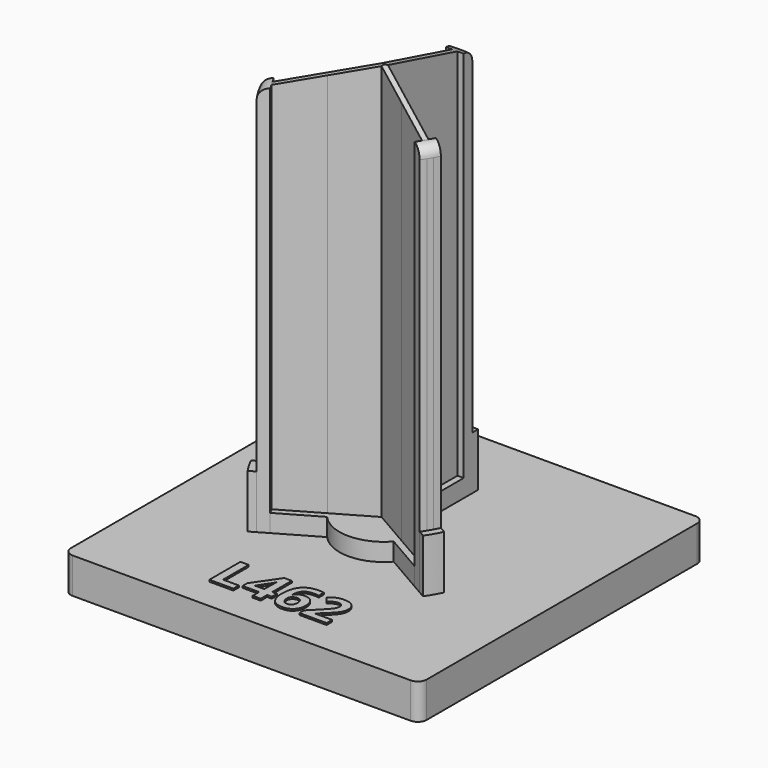
from build123d import *

# Parameters (mm, degrees)
F0_R         = 3.5
F0_R_2       = 1.75
F1_DEPTH     = 10
F2_DEPTH     = 220
F3_DEPTH     = 235
F4_T4_DEPTH  = 293.7329049929
F4_T9_DEPTH  = 293.7329049929
F4_T14_DEPTH = 293.7329049929
F5_T2_ANGLE  = 40.9393595263
F5_T4_ANGLE  = 40.9393595263
F5_T6_ANGLE  = 40.9393595263
F6_DEPTH     = 3
F7_DEPTH     = 30
F8_W         = 200
F8_H         = 200
F9_DEPTH     = 20
F10_R        = 5
F0_TEXT_SIZE = 30.5555555556
F11_DEPTH    = 1


# Not quite as in the source:
# - a fillet or chamfer that OpenCascade refuses, or shapes differently, is made with other operations: its cross-section is extruded or revolved along the edge and cut away or added
# - a feature names something its author has since deleted; it is built from what else it names
# - Text() gives the source's letters only with a copy of the font that has no kerning and outlines rounded to 1/6400 em; it was checked with that copy


with BuildPart() as f1:
    # F0 (on Top) → F1 (new body)
    with BuildSketch(Plane.XY):
        with BuildLine():
            ThreePointArc((25, 0), (19.364916731, 15.8113883008), (5, 24.4948974278))
            ThreePointArc((5, 24.4948974278), (3.2581304855, 24.7867824806), (1.5, 24.9549594269))
            Line((1.5, 24.9549594269), (1.5, 0.8660254038))
            Line((1.5, 0.8660254038), (22.3616288141, -11.1784416078))
            ThreePointArc((22.3616288141, -11.1784416078), (23.095048549, -9.571767471), (23.7132034356, -7.917321695))
            ThreePointArc((23.7132034356, -7.917321695), (24.6762039817, -4.0106055721), (25, 0))
        make_face()
        with Locations((11.9308144071, 6.8882589096)):
            Circle(F0_R, mode=Mode.SUBTRACT)
        with BuildLine():
            Line((5, 24.4948974278), (5, 49.7493718553))
            Line((5, 49.7493718553), (1.5, 49.7493718553))
            Line((1.5, 49.7493718553), (1.5, 24.9549594269))
            ThreePointArc((1.5, 24.9549594269), (3.2581304855, 24.7867824806), (5, 24.4948974278))
        make_face()
        with BuildLine():
            Line((43.834219849, -23.575647822), (45.584219849, -20.5445589087))
            Line((45.584219849, -20.5445589087), (23.7132034356, -7.917321695))
            ThreePointArc((23.7132034356, -7.917321695), (23.095048549, -9.571767471), (22.3616288141, -11.1784416078))
            Line((22.3616288141, -11.1784416078), (43.834219849, -23.575647822))
        make_face()
        with Locations((11.9308144071, 6.8882589096)):
            Circle(F0_R)
        with Locations((11.9308144071, 6.8882589096)):
            Circle(F0_R_2, mode=Mode.SUBTRACT)
        with Locations((11.9308144071, 6.8882589096)):
            Circle(F0_R_2)
    extrude(amount=F1_DEPTH)



with BuildPart() as f1b:
    # F0 (on Top) → F1, piece 2 (new body)
    with BuildSketch(Plane.XY):
        with BuildLine():
            Line((-1.5, 49.7493718553), (-5, 49.7493718553))
            Line((-5, 49.7493718553), (-5, 24.4948974278))
            ThreePointArc((-5, 24.4948974278), (-3.2581304855, 24.7867824806), (-1.5, 24.9549594269))
            Line((-1.5, 24.9549594269), (-1.5, 49.7493718553))
        make_face()
        with BuildLine():
            Line((-23.7132034356, -7.917321695), (-45.584219849, -20.5445589087))
            Line((-45.584219849, -20.5445589087), (-43.834219849, -23.575647822))
            Line((-43.834219849, -23.575647822), (-22.3616288141, -11.1784416078))
            ThreePointArc((-22.3616288141, -11.1784416078), (-23.095048549, -9.571767471), (-23.7132034356, -7.917321695))
        make_face()
        with BuildLine():
            ThreePointArc((-1.5, 24.9549594269), (-3.2581304855, 24.7867824806), (-5, 24.4948974278))
            ThreePointArc((-5, 24.4948974278), (-21.6506350946, 12.5), (-23.7132034356, -7.917321695))
            ThreePointArc((-23.7132034356, -7.917321695), (-23.095048549, -9.571767471), (-22.3616288141, -11.1784416078))
            Line((-22.3616288141, -11.1784416078), (-1.5, 0.8660254038))
            Line((-1.5, 0.8660254038), (-1.5, 24.9549594269))
        make_face()
        with Locations((-11.9308144071, 6.8882589096)):
            Circle(F0_R, mode=Mode.SUBTRACT)
        with Locations((-11.9308144071, 6.8882589096)):
            Circle(F0_R)
        with Locations((-11.9308144071, 6.8882589096)):
            Circle(F0_R_2, mode=Mode.SUBTRACT)
        with Locations((-11.9308144071, 6.8882589096)):
            Circle(F0_R_2)
    extrude(amount=F1_DEPTH)


with BuildPart() as f1c:
    # F0 (on Top) → F1, piece 3 (new body)
    with BuildSketch(Plane.XY):
        with BuildLine():
            ThreePointArc((-18.7132034356, -16.5775757328), (0, -25), (18.7132034356, -16.5775757328))
            ThreePointArc((18.7132034356, -16.5775757328), (19.8369180635, -15.2150150096), (20.8616288141, -13.7765178191))
            Line((20.8616288141, -13.7765178191), (0, -1.7320508076))
            Line((0, -1.7320508076), (-20.8616288141, -13.7765178191))
            ThreePointArc((-20.8616288141, -13.7765178191), (-19.8369180635, -15.2150150096), (-18.7132034356, -16.5775757328))
        make_face()
        with Locations((0, -13.7765178191)):
            Circle(F0_R, mode=Mode.SUBTRACT)
        with BuildLine():
            Line((18.7132034356, -16.5775757328), (40.584219849, -29.2048129466))
            Line((40.584219849, -29.2048129466), (42.334219849, -26.1737240333))
            Line((42.334219849, -26.1737240333), (20.8616288141, -13.7765178191))
            ThreePointArc((20.8616288141, -13.7765178191), (19.8369180635, -15.2150150096), (18.7132034356, -16.5775757328))
        make_face()
        with BuildLine():
            Line((-42.334219849, -26.1737240333), (-40.584219849, -29.2048129466))
            Line((-40.584219849, -29.2048129466), (-18.7132034356, -16.5775757328))
            ThreePointArc((-18.7132034356, -16.5775757328), (-19.8369180635, -15.2150150096), (-20.8616288141, -13.7765178191))
            Line((-20.8616288141, -13.7765178191), (-42.334219849, -26.1737240333))
        make_face()
        with Locations((0, -13.7765178191)):
            Circle(F0_R)
        with Locations((0, -13.7765178191)):
            Circle(F0_R_2, mode=Mode.SUBTRACT)
        with Locations((0, -13.7765178191)):
            Circle(F0_R_2)
    extrude(amount=F1_DEPTH)


with BuildPart() as f1_1:
    add(f1.part)

    add(f1b.part)  # F2 merges F1b

    add(f1c.part)  # F2 merges F1c
    # F0 (on Top) → F2 (join)
    with BuildSketch(Plane.XY):
        with BuildLine():
            Line((5, 49.7493718553), (5, 55.7763390695))
            ThreePointArc((5, 55.7763390695), (3.2515934535, 55.9055197634), (1.5, 55.9799071096))
            Line((1.5, 55.9799071096), (1.5, 49.7493718553))
            Line((1.5, 49.7493718553), (5, 49.7493718553))
        make_face()
        with BuildLine():
            ThreePointArc((-1.5, 55.9799071096), (-3.2515934535, 55.9055197634), (-5, 55.7763390695))
            Line((-5, 55.7763390695), (-5, 49.7493718553))
            Line((-5, 49.7493718553), (-1.5, 49.7493718553))
            Line((-1.5, 49.7493718553), (-1.5, 55.9799071096))
        make_face()
        with BuildLine():
            ThreePointArc((-47.7300216584, -29.2889916605), (-46.7898036001, -30.7687224152), (-45.8037265643, -32.2182965537))
            Line((-45.8037265643, -32.2182965537), (-40.584219849, -29.2048129466))
            Line((-40.584219849, -29.2048129466), (-42.334219849, -26.1737240333))
            Line((-42.334219849, -26.1737240333), (-47.7300216584, -29.2889916605))
        make_face()
        with BuildLine():
            Line((-45.584219849, -20.5445589087), (-50.8037265643, -23.5580425158))
            ThreePointArc((-50.8037265643, -23.5580425158), (-50.0413970536, -25.1367973482), (-49.2300216584, -26.6909154491))
            Line((-49.2300216584, -26.6909154491), (-43.834219849, -23.575647822))
            Line((-43.834219849, -23.575647822), (-45.584219849, -20.5445589087))
        make_face()
        with BuildLine():
            Line((40.584219849, -29.2048129466), (45.8037265643, -32.2182965537))
            ThreePointArc((45.8037265643, -32.2182965537), (46.7898036001, -30.7687224152), (47.7300216584, -29.2889916605))
            Line((47.7300216584, -29.2889916605), (42.334219849, -26.1737240333))
            Line((42.334219849, -26.1737240333), (40.584219849, -29.2048129466))
        make_face()
        with BuildLine():
            ThreePointArc((49.2300216584, -26.6909154491), (50.0413970536, -25.1367973482), (50.8037265643, -23.5580425158))
            Line((50.8037265643, -23.5580425158), (45.584219849, -20.5445589087))
            Line((45.584219849, -20.5445589087), (43.834219849, -23.575647822))
            Line((43.834219849, -23.575647822), (49.2300216584, -26.6909154491))
        make_face()
        with BuildLine():
            Line((-43.834219849, -23.575647822), (-49.2300216584, -26.6909154491))
            ThreePointArc((-49.2300216584, -26.6909154491), (-48.4974226119, -28), (-47.7300216584, -29.2889916605))
            Line((-47.7300216584, -29.2889916605), (-42.334219849, -26.1737240333))
            Line((-42.334219849, -26.1737240333), (-43.834219849, -23.575647822))
        make_face()
        with BuildLine():
            ThreePointArc((47.7300216584, -29.2889916605), (48.4974226119, -28), (49.2300216584, -26.6909154491))
            Line((49.2300216584, -26.6909154491), (43.834219849, -23.575647822))
            Line((43.834219849, -23.575647822), (42.334219849, -26.1737240333))
            Line((42.334219849, -26.1737240333), (47.7300216584, -29.2889916605))
        make_face()
        with BuildLine():
            Line((1.5, 49.7493718553), (1.5, 55.9799071096))
            ThreePointArc((1.5, 55.9799071096), (0, 56), (-1.5, 55.9799071096))
            Line((-1.5, 55.9799071096), (-1.5, 49.7493718553))
            Line((-1.5, 49.7493718553), (1.5, 49.7493718553))
        make_face()
    extrude(amount=F2_DEPTH)

    # F0 (on Top) → F3 (join)
    with BuildSketch(Plane.XY):
        with BuildLine():
            Line((1.5, 0.8660254038), (1.5, 24.9549594269))
            ThreePointArc((1.5, 24.9549594269), (0, 25), (-1.5, 24.9549594269))
            Line((-1.5, 24.9549594269), (-1.5, 0.8660254038))
            Line((-1.5, 0.8660254038), (-22.3616288141, -11.1784416078))
            ThreePointArc((-22.3616288141, -11.1784416078), (-21.6506350946, -12.5), (-20.8616288141, -13.7765178191))
            Line((-20.8616288141, -13.7765178191), (0, -1.7320508076))
            Line((0, -1.7320508076), (20.8616288141, -13.7765178191))
            ThreePointArc((20.8616288141, -13.7765178191), (21.6506350946, -12.5), (22.3616288141, -11.1784416078))
            Line((22.3616288141, -11.1784416078), (1.5, 0.8660254038))
        make_face()
        with BuildLine():
            Line((1.5, 24.9549594269), (1.5, 49.7493718553))
            Line((1.5, 49.7493718553), (-1.5, 49.7493718553))
            Line((-1.5, 49.7493718553), (-1.5, 24.9549594269))
            ThreePointArc((-1.5, 24.9549594269), (0, 25), (1.5, 24.9549594269))
        make_face()
        with BuildLine():
            Line((-22.3616288141, -11.1784416078), (-43.834219849, -23.575647822))
            Line((-43.834219849, -23.575647822), (-42.334219849, -26.1737240333))
            Line((-42.334219849, -26.1737240333), (-20.8616288141, -13.7765178191))
            ThreePointArc((-20.8616288141, -13.7765178191), (-21.6506350946, -12.5), (-22.3616288141, -11.1784416078))
        make_face()
        with BuildLine():
            Line((42.334219849, -26.1737240333), (43.834219849, -23.575647822))
            Line((43.834219849, -23.575647822), (22.3616288141, -11.1784416078))
            ThreePointArc((22.3616288141, -11.1784416078), (21.6506350946, -12.5), (20.8616288141, -13.7765178191))
            Line((20.8616288141, -13.7765178191), (42.334219849, -26.1737240333))
        make_face()
    extrude(amount=F3_DEPTH)

    # F4: chamfer of 15 x 55.9807621135 on 3 edges, made by hand


with BuildPart() as f4_tool2:
    # F4_s3 → F4_t4 (new body)
    with BuildSketch(Plane(origin=(-73.4332262482, -127.1900788256, 0), x_dir=(0, 0, 1), z_dir=(0.5, 0.8660254038, 0))):
        Polygon((220, 49.7493718553), (235, -6.2313902582), (235, 49.7493718553), align=None)
    extrude(amount=F4_T4_DEPTH)

    split(bisect_by=Plane.XY.offset(220), keep=Keep.TOP)


with BuildPart() as f1_2:
    add(f1_1.part)

    # F4_t1: cut F4_tool2
    add(f4_tool2.part, mode=Mode.SUBTRACT)


with BuildPart() as f4_tool7:
    # F4_s8 → F4_t9 (new body)
    with BuildSketch(Plane(origin=(-73.4332262482, 127.1900788256, 0), x_dir=(0, 0, 1), z_dir=(0.5, -0.8660254038, 0))):
        Polygon((235, -6.2313902582), (220, 49.7493718553), (235, 49.7493718553), align=None)
    extrude(amount=F4_T9_DEPTH)

    split(bisect_by=Plane.XY.offset(220), keep=Keep.TOP)


with BuildPart() as f1_3:
    add(f1_2.part)

    # F4_t6: cut F4_tool7
    add(f4_tool7.part, mode=Mode.SUBTRACT)


with BuildPart() as f4_tool12:
    # F4_s13 → F4_t14 (new body)
    with BuildSketch(Plane.YZ.offset(146.8664524965)):
        Polygon((-6.2313902582, 235), (49.7493718553, 220), (49.7493718553, 235), align=None)
    extrude(amount=-F4_T14_DEPTH)

    split(bisect_by=Plane.XY.offset(220), keep=Keep.TOP)


with BuildPart() as f1_4:
    add(f1_3.part)

    # F4_t11: cut F4_tool12
    add(f4_tool12.part, mode=Mode.SUBTRACT)

    # F5: fillet of radius 6 on 3 edges, made by hand

    # F5_s1 → F5_t2 (revolve, cut)
    with BuildSketch(Plane(origin=(0, 0, 0), x_dir=(0, 0, 1), z_dir=(-0.7712878704, -0.6364864656, 0))):
        with BuildLine():
            ThreePointArc((220, -50), (218.2426406871, -54.2426406871), (214, -56))
            Line((214, -56), (220, -56))
            Line((220, -56), (220, -50))
        make_face()
    revolve(axis=Axis((0, 0, 220), (0, 0, 1)), revolution_arc=F5_T2_ANGLE, mode=Mode.SUBTRACT)

    # F5_s3 → F5_t4 (revolve, cut)
    with BuildSketch(Plane(origin=(0, 0, 0), x_dir=(0, 0, 1), z_dir=(0.9368573836, -0.3497116566, 0))):
        with BuildLine():
            ThreePointArc((214, -56), (218.2426406871, -54.2426406871), (220, -50))
            Line((220, -50), (220, -56))
            Line((220, -56), (214, -56))
        make_face()
    revolve(axis=Axis((0, 0, 220), (0, 0, 1)), revolution_arc=F5_T4_ANGLE, mode=Mode.SUBTRACT)

    # F5_s5 → F5_t6 (revolve, cut)
    with BuildSketch(Plane(origin=(0, 0, 0), x_dir=(0, 0, 1), z_dir=(-0.1655695132, 0.9861981222, 0))):
        with BuildLine():
            ThreePointArc((214, -56), (218.2426406871, -54.2426406871), (220, -50))
            Line((220, -50), (220, -56))
            Line((220, -56), (214, -56))
        make_face()
    revolve(axis=Axis((0, 0, 220), (0, 0, 1)), revolution_arc=F5_T6_ANGLE, mode=Mode.SUBTRACT)

    # F0 (on Top) → F6 (join)
    with BuildSketch(Plane.XY):
        with Locations((-11.9308144071, 6.8882589096)):
            Circle(F0_R)
        with Locations((-11.9308144071, 6.8882589096)):
            Circle(F0_R_2, mode=Mode.SUBTRACT)
        with Locations((0, -13.7765178191)):
            Circle(F0_R)
        with Locations((0, -13.7765178191)):
            Circle(F0_R_2, mode=Mode.SUBTRACT)
        with Locations((11.9308144071, 6.8882589096)):
            Circle(F0_R)
        with Locations((11.9308144071, 6.8882589096)):
            Circle(F0_R_2, mode=Mode.SUBTRACT)
    extrude(amount=F6_DEPTH)

    # F0 (on Top) → F7 (join)
    with BuildSketch(Plane.XY):
        with BuildLine():
            Line((-50.8037265643, -23.5580425158), (-54.280787943, -25.5655248388))
            ThreePointArc((-54.280787943, -25.5655248388), (-51.9615242271, -30), (-49.280787943, -34.2257788767))
            Line((-49.280787943, -34.2257788767), (-45.8037265643, -32.2182965537))
            ThreePointArc((-45.8037265643, -32.2182965537), (-46.7898036001, -30.7687224152), (-47.7300216584, -29.2889916605))
            ThreePointArc((-47.7300216584, -29.2889916605), (-48.4974226119, -28), (-49.2300216584, -26.6909154491))
            ThreePointArc((-49.2300216584, -26.6909154491), (-50.0413970536, -25.1367973482), (-50.8037265643, -23.5580425158))
        make_face()
        with BuildLine():
            ThreePointArc((49.280787943, -34.2257788767), (51.9615242271, -30), (54.280787943, -25.5655248388))
            Line((54.280787943, -25.5655248388), (50.8037265643, -23.5580425158))
            ThreePointArc((50.8037265643, -23.5580425158), (50.0413970536, -25.1367973482), (49.2300216584, -26.6909154491))
            ThreePointArc((49.2300216584, -26.6909154491), (48.4974226119, -28), (47.7300216584, -29.2889916605))
            ThreePointArc((47.7300216584, -29.2889916605), (46.7898036001, -30.7687224152), (45.8037265643, -32.2182965537))
            Line((45.8037265643, -32.2182965537), (49.280787943, -34.2257788767))
        make_face()
        with BuildLine():
            Line((5, 55.7763390695), (5, 59.7913037155))
            ThreePointArc((5, 59.7913037155), (0, 60), (-5, 59.7913037155))
            Line((-5, 59.7913037155), (-5, 55.7763390695))
            ThreePointArc((-5, 55.7763390695), (-3.2515934535, 55.9055197634), (-1.5, 55.9799071096))
            ThreePointArc((-1.5, 55.9799071096), (0, 56), (1.5, 55.9799071096))
            ThreePointArc((1.5, 55.9799071096), (3.2515934535, 55.9055197634), (5, 55.7763390695))
        make_face()
    extrude(amount=F7_DEPTH)

    # F8 (on Top) → F9 (join)
    with BuildSketch(Plane.XY):
        Rectangle(F8_W, F8_H)
    extrude(amount=-F9_DEPTH)

    # F10
    f10_edges = [f1_4.edges().sort_by_distance(p)[0] for p in [
        (-100, -100, -10),
        (100, -100, -10),
        (100, 100, -10),
        (-100, 100, -10),
    ]]
    fillet(f10_edges, radius=F10_R)

    # F0 (on Top) → F11 (join)
    with BuildSketch(Plane.XY):
        with Locations((-35.298828125, -82)):
            Text('L462', F0_TEXT_SIZE, font='Open Sans', font_style=FontStyle.BOLD, text_align=(TextAlign.LEFT, TextAlign.BOTTOM))
    extrude(amount=F11_DEPTH)


solid = f1_4.part
